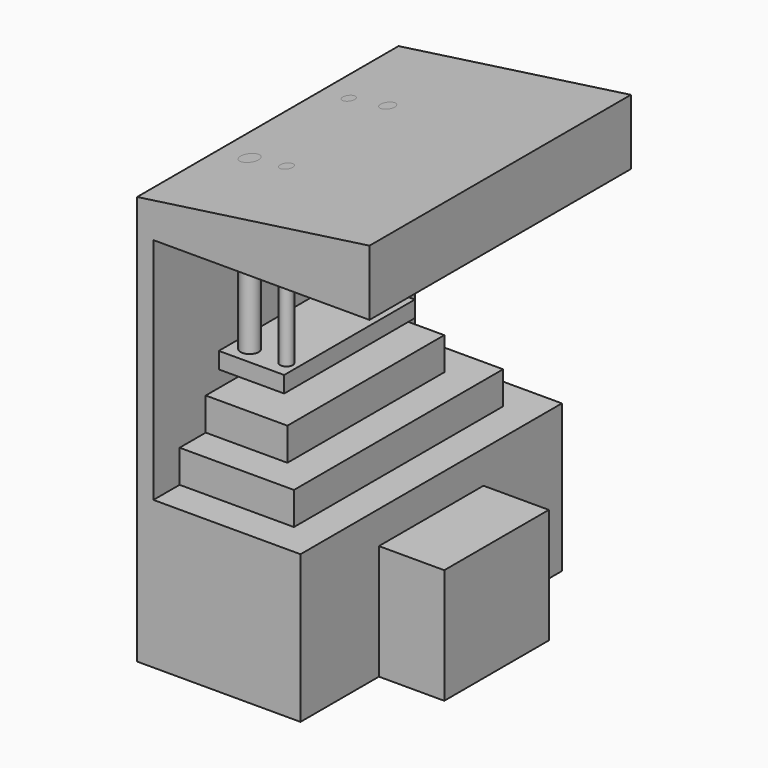
from build123d import *

# Parameters (mm, degrees)
F1_DEPTH  = 12.7
F0_W      = 5.08
F0_H      = 8.9359007079
F2_DEPTH  = 5.08
F3_DEPTH  = 10.16
F0_W_2    = 6.35
F0_H_2    = 2.54
F4_DEPTH  = 7.62
F8_W      = 5.08
F8_H      = 12.7
F9_DEPTH  = 1.27
F10_R     = 0.6993385281
F11_REACH = 17.2190280622
F10_R_2   = 0.4846158618
F10_R_3   = 0.4668021957
F10_R_4   = 0.550131889


with BuildPart() as f1:
    # F0 (on Front) → F1 (new body, symmetric)
    with BuildSketch(Plane.XZ):
        Polygon((0, 31.7959007079), (0, 0), (12.7, 0), (12.7, 8.9359007079), (12.7, 11.4759007079), (10.16, 11.4759007079), (1.27, 11.4759007079), (1.27, 14.0159007079), (1.27, 16.5559007079), (1.27, 29.2559007079), (18.063576892, 29.2559007079), (18.063576892, 34.3359007079), align=None)
    extrude(amount=F1_DEPTH, both=True)

    # F0 (on Front) → F2 (join, symmetric)
    with BuildSketch(Plane.XZ):
        with Locations((15.24, 4.467950354)):
            Rectangle(F0_W, F0_H)
    extrude(amount=F2_DEPTH, both=True)

    # F0 (on Front) → F3 (join, symmetric)
    with BuildSketch(Plane.XZ):
        Polygon((1.27, 11.4759007079), (10.16, 11.4759007079), (10.16, 14.0159007079), (7.62, 14.0159007079), (1.27, 14.0159007079), align=None)
    extrude(amount=F3_DEPTH, both=True)

    # F0 (on Front) → F4 (join, symmetric)
    with BuildSketch(Plane.XZ):
        with Locations((4.445, 15.2859007079)):
            Rectangle(F0_W_2, F0_H_2)
    extrude(amount=F4_DEPTH, both=True)

    # F8 (on offset) → F9 (join)
    with BuildSketch(Plane.XY.offset(17.8259007079)):
        with Locations((3.81, 0)):
            Rectangle(F8_W, F8_H)
    extrude(amount=F9_DEPTH)


with BuildPart() as f6:
    # F5 (on Front) → F6 (revolve)
    with BuildSketch(Plane.XZ):
        with BuildLine():
            ThreePointArc((6.858, 28.5420352743), (3.8318670551, 27.2097778537), (1.6425333333, 24.7320352743))
            Line((1.6425333333, 24.7320352743), (6.858, 24.7320352743))
            Line((6.858, 24.7320352743), (6.858, 28.5420352743))
        make_face()
    revolve(axis=Axis((6.858, 0, 28.8225058466), (0, 0, -1)))


with BuildPart() as f11:
    f11_end = f1.part.faces().sort_by_distance((9.031788446, 0, 33.0659007079))[0]
    # F10 (on face) → F11 (new body, up to a face of F1 that its end follows)
    with BuildSketch(Plane.XY.offset(19.0959007079)):
        with Locations((2.5612919126, -4.9697342329)):
            Circle(F10_R)
    f11_long = extrude(amount=F11_REACH, mode=Mode.PRIVATE)
    add(split(f11_long, bisect_by=f11_end, keep=Keep.BOTTOM, mode=Mode.PRIVATE))


with BuildPart() as f11b:
    f11_2_end = f1.part.faces().sort_by_distance((9.031788446, 0, 33.0659007079))[0]
    # F10 (on face) → F11, piece 2 (new body, up to a face of F1 that its end follows)
    with BuildSketch(Plane.XY.offset(19.0959007079)):
        with Locations((5.4644043557, -5.0189397298)):
            Circle(F10_R_2)
    f11_2_long = extrude(amount=F11_REACH, mode=Mode.PRIVATE)
    add(split(f11_2_long, bisect_by=f11_2_end, keep=Keep.BOTTOM, mode=Mode.PRIVATE))


with BuildPart() as f11c:
    f11_3_end = f1.part.faces().sort_by_distance((9.031788446, 0, 33.0659007079))[0]
    # F10 (on face) → F11, piece 3 (new body, up to a face of F1 that its end follows)
    with BuildSketch(Plane.XY.offset(19.0959007079)):
        with Locations((2.3152653594, 4.9697356299)):
            Circle(F10_R_3)
    f11_3_long = extrude(amount=F11_REACH, mode=Mode.PRIVATE)
    add(split(f11_3_long, bisect_by=f11_3_end, keep=Keep.BOTTOM, mode=Mode.PRIVATE))


with BuildPart() as f11d:
    f11_4_end = f1.part.faces().sort_by_distance((9.031788446, 0, 33.0659007079))[0]
    # F10 (on face) → F11, piece 4 (new body, up to a face of F1 that its end follows)
    with BuildSketch(Plane.XY.offset(19.0959007079)):
        with Locations((5.2675828338, 5.0681466237)):
            Circle(F10_R_4)
    f11_4_long = extrude(amount=F11_REACH, mode=Mode.PRIVATE)
    add(split(f11_4_long, bisect_by=f11_4_end, keep=Keep.BOTTOM, mode=Mode.PRIVATE))


solid = Compound([f1.part, f6.part, f11.part, f11b.part, f11c.part, f11d.part])
